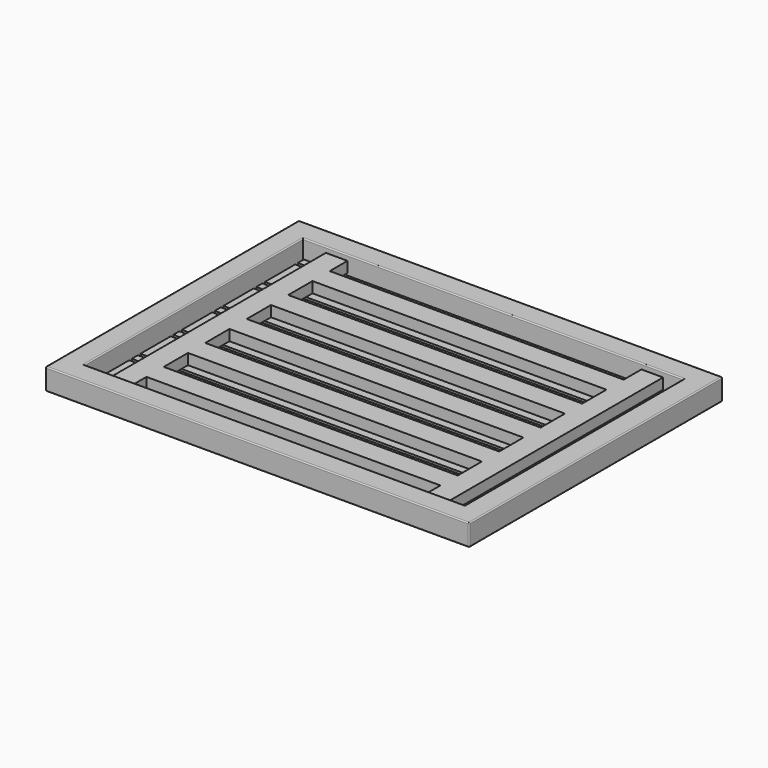
from build123d import *

# Parameters (mm, degrees)
F0_W     = 1960
F0_H     = 1465
F0_W_2   = 1760
F0_H_2   = 1265
F1_DEPTH = 100
F2_DEPTH = 25
F0_W_3   = 1730
F0_H_3   = 175
F0_H_4   = 35
F3_R     = 5
F4_R     = 5
F5_W     = 1360
F5_H     = 140
F6_DEPTH = 50


# Not quite as in the source:
# - a feature names something its author has since deleted; it is built from what else it names


with BuildPart() as f1:
    # F0 (on Top) → F1 (new body)
    with BuildSketch(Plane.XY):
        with Locations((980, 732.5)):
            Rectangle(F0_W, F0_H)
        with Locations((980, 732.5)):
            Rectangle(F0_W_2, F0_H_2, mode=Mode.SUBTRACT)
    extrude(amount=F1_DEPTH)

    # F0 (on Top) → F2 (join)
    with BuildSketch(Plane.XY):
        with Locations((980, 732.5)):
            Rectangle(F0_W, F0_H)
        with Locations((980, 732.5)):
            Rectangle(F0_W_2, F0_H_2, mode=Mode.SUBTRACT)
    extrude(amount=F2_DEPTH)

    # F3
    f3_edges = [f1.edges().sort_by_distance(p)[0] for p in [
        (980, 1365, 100),
        (100, 732.5, 100),
        (980, 100, 100),
        (1860, 732.5, 100),
    ]]
    fillet(f3_edges, radius=F3_R)

    # F4
    f4_edges = [f1.edges().sort_by_distance(p)[0] for p in [
        (980, 1465, 100),
        (0, 732.5, 100),
        (1960, 732.5, 100),
        (980, 0, 100),
        (1960, 0, 50),
        (0, 0, 50),
        (980, 0, 0),
        (0, 732.5, 0),
        (0, 1465, 50),
        (980, 1465, 0),
        (1960, 1465, 50),
        (1960, 732.5, 0),
        (100, 732.5, 0),
        (980, 1365, 0),
        (980, 100, 0),
        (1860, 732.5, 0),
    ]]
    fillet(f4_edges, radius=F4_R)


with BuildPart() as f2:
    # F0 (on Top) → F2, piece 2 (new body)
    with BuildSketch(Plane.XY):
        with Locations((980, 1212.5)):
            Rectangle(F0_W_3, F0_H_3)
    extrude(amount=F2_DEPTH)


with BuildPart() as f2b:
    # F0 (on Top) → F2, piece 3 (new body)
    with BuildSketch(Plane.XY):
        with Locations((980, 972.5)):
            Rectangle(F0_W_3, F0_H_3)
    extrude(amount=F2_DEPTH)


with BuildPart() as f2c:
    # F0 (on Top) → F2, piece 4 (new body)
    with BuildSketch(Plane.XY):
        with Locations((980, 732.5)):
            Rectangle(F0_W_3, F0_H_3)
    extrude(amount=F2_DEPTH)


with BuildPart() as f2d:
    # F0 (on Top) → F2, piece 5 (new body)
    with BuildSketch(Plane.XY):
        with Locations((980, 492.5)):
            Rectangle(F0_W_3, F0_H_3)
    extrude(amount=F2_DEPTH)


with BuildPart() as f2e:
    # F0 (on Top) → F2, piece 6 (new body)
    with BuildSketch(Plane.XY):
        with Locations((980, 252.5)):
            Rectangle(F0_W_3, F0_H_3)
    extrude(amount=F2_DEPTH)


with BuildPart() as f2f:
    # F0 (on Top) → F2, piece 7 (new body)
    with BuildSketch(Plane.XY):
        with Locations((980, 132.5)):
            Rectangle(F0_W_3, F0_H_4)
    extrude(amount=F2_DEPTH)


with BuildPart() as f2g:
    # F0 (on Top) → F2, piece 8 (new body)
    with BuildSketch(Plane.XY):
        with Locations((980, 372.5)):
            Rectangle(F0_W_3, F0_H_4)
    extrude(amount=F2_DEPTH)


with BuildPart() as f2h:
    # F0 (on Top) → F2, piece 9 (new body)
    with BuildSketch(Plane.XY):
        with Locations((980, 612.5)):
            Rectangle(F0_W_3, F0_H_4)
    extrude(amount=F2_DEPTH)


with BuildPart() as f2i:
    # F0 (on Top) → F2, piece 10 (new body)
    with BuildSketch(Plane.XY):
        with Locations((980, 852.5)):
            Rectangle(F0_W_3, F0_H_4)
    extrude(amount=F2_DEPTH)


with BuildPart() as f2j:
    # F0 (on Top) → F2, piece 11 (new body)
    with BuildSketch(Plane.XY):
        with Locations((980, 1092.5)):
            Rectangle(F0_W_3, F0_H_4)
    extrude(amount=F2_DEPTH)


with BuildPart() as f2k:
    # F0 (on Top) → F2, piece 12 (new body)
    with BuildSketch(Plane.XY):
        with Locations((980, 1332.5)):
            Rectangle(F0_W_3, F0_H_4)
    extrude(amount=F2_DEPTH)


with BuildPart() as f6:
    # F5 (on face) → F6 (new body)
    with BuildSketch(Plane.XY.offset(25)):
        Polygon((205, 1365), (205, 100), (305, 100), (305, 202.5), (1665, 202.5), (1665, 100), (1765, 100), (1765, 1365), (1665, 1365), (1665, 1262.5), (305, 1262.5), (305, 1365), align=None)
        with Locations((985, 372.5)):
            Rectangle(F5_W, F5_H, mode=Mode.SUBTRACT)
        with Locations((985, 612.5)):
            Rectangle(F5_W, F5_H, mode=Mode.SUBTRACT)
        with Locations((985, 852.5)):
            Rectangle(F5_W, F5_H, mode=Mode.SUBTRACT)
        with Locations((985, 1092.5)):
            Rectangle(F5_W, F5_H, mode=Mode.SUBTRACT)
    extrude(amount=F6_DEPTH)


solid = Compound([f1.part, f2.part, f2b.part, f2c.part, f2d.part, f2e.part, f2f.part, f2g.part, f2h.part, f2i.part, f2j.part, f2k.part, f6.part])
